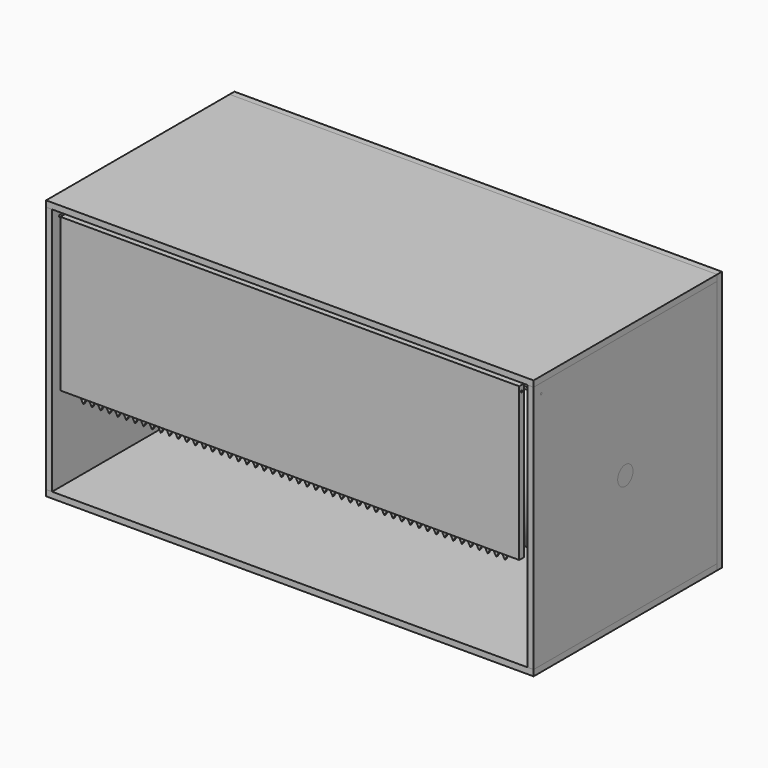
from build123d import *

# Parameters (mm, degrees)
F1_W           = 255
F1_H           = 120
F2_DEPTH       = 3.15
F3_W           = 120
F3_H           = 130
F4_DEPTH       = 3.15
F7_W           = 255
F7_H           = 136.3
F8_DEPTH       = 3.15
F11_R          = 42.8170068392
F11_R_2        = 11.8370629582
F12_DEPTH      = 115
F12_DEPTH_BACK = 115
F13_W          = 240
F13_H          = 80
F14_DEPTH      = 3.15
F16_DEPTH      = 1
F17_R          = 5
F17_R_2        = 0.5
F18_DEPTH      = 255.001
F19_R          = 5
F20_DEPTH      = 255
F19_R_2        = 0.5
F21_R          = 0.5
F22_DEPTH      = 247.501


with BuildPart() as f2:
    # F1 (on Top) → F2 (new body)
    with BuildSketch(Plane.XY):
        with Locations((127.5, 60)):
            Rectangle(F1_W, F1_H)
    extrude(amount=F2_DEPTH)


with BuildPart() as f4:
    # F3 (on face) → F4 (new body)
    with BuildSketch(Plane(origin=(0, 0, 0), x_dir=(0, -1, 0), z_dir=(-1, 0, 0))):
        with Locations((-60, 68.15)):
            Rectangle(F3_W, F3_H)
    extrude(amount=-F4_DEPTH)


with BuildPart() as f5_1:
    # F5: copy of F2
    add(f2.part.moved(Location((0, 0, 133.15))))


with BuildPart() as f6_1:
    # F6: copy of F4
    add(f4.part.moved(Location((251.85, 0, 0))))


with BuildPart() as f8:
    # F7 (on face) → F8 (new body)
    with BuildSketch(Plane(origin=(0, 120, 0), x_dir=(-1, 0, 0), z_dir=(0, 1, 0))):
        with Locations((-127.5, 68.15)):
            Rectangle(F7_W, F7_H)
    extrude(amount=F8_DEPTH)


with BuildPart() as f12:
    # F11 (on plane+point) → F12 (new body, two sides)
    with BuildSketch(Plane.YZ.offset(127.5)) as f12_sk:
        with Locations((62.5, 68.15)):
            Circle(F11_R)
        with Locations((62.5, 68.15)):
            Circle(F11_R_2, mode=Mode.SUBTRACT)
    extrude(amount=F12_DEPTH)
    extrude(f12_sk.sketch, amount=-F12_DEPTH_BACK)


with BuildPart() as f14:
    # F13 (on face) → F14 (new body)
    with BuildSketch(Plane.XZ):
        with Locations((127.5, 91.15)):
            Rectangle(F13_W, F13_H)
    extrude(amount=-F14_DEPTH)

    # F21 (on face) → F22 (cut, through all)
    with BuildSketch(Plane.YZ.offset(247.5)):
        with Locations((1.575, 128.15)):
            Circle(F21_R)
    extrude(amount=-F22_DEPTH, mode=Mode.SUBTRACT)


with BuildPart() as f16:
    # F15 (on face) → F16 (new body)
    with BuildSketch(Plane(origin=(0, 3.15, 0), x_dir=(-1, 0, 0), z_dir=(0, 1, 0))):
        Polygon((-231.0417766441, 51.15), (-234.8456242214, 51.15), (-235.1937004328, 50.547114317), (-232.9437004328, 46.65), (-230.6937004328, 50.547114317), align=None)
        Polygon((-235.1937004328, 50.547114317), (-234.8456242214, 51.15), (-235.5417766441, 51.15), align=None)
        Polygon((-235.5417766441, 51.15), (-234.8456242214, 51.15), (-231.0417766441, 51.15), (-230.3456242214, 51.15), (-226.5417766441, 51.15), (-225.8456242214, 51.15), (-222.0417766441, 51.15), (-221.3456242214, 51.15), (-217.5417766441, 51.15), (-216.8456242214, 51.15), (-213.0417766441, 51.15), (-212.3456242214, 51.15), (-208.5417766441, 51.15), (-207.8456242214, 51.15), (-204.0417766441, 51.15), (-203.3456242214, 51.15), (-199.5417766441, 51.15), (-198.8456242214, 51.15), (-195.0417766441, 51.15), (-194.3456242214, 51.15), (-190.5417766441, 51.15), (-189.8456242214, 51.15), (-186.0417766441, 51.15), (-185.3456242214, 51.15), (-181.5417766441, 51.15), (-180.8456242214, 51.15), (-177.0417766441, 51.15), (-176.3456242214, 51.15), (-172.5417766441, 51.15), (-171.8456242214, 51.15), (-168.0417766441, 51.15), (-167.3456242214, 51.15), (-163.5417766441, 51.15), (-162.8456242214, 51.15), (-159.0417766441, 51.15), (-158.3456242214, 51.15), (-154.5417766441, 51.15), (-153.8456242214, 51.15), (-150.0417766441, 51.15), (-149.3456242214, 51.15), (-145.5417766441, 51.15), (-144.8456242214, 51.15), (-141.0417766441, 51.15), (-140.3456242214, 51.15), (-136.5417766441, 51.15), (-135.8456242214, 51.15), (-132.0417766441, 51.15), (-131.3456242214, 51.15), (-127.5417766441, 51.15), (-126.8456242214, 51.15), (-123.0417766441, 51.15), (-122.3456242214, 51.15), (-118.5417766441, 51.15), (-117.8456242214, 51.15), (-114.0417766441, 51.15), (-113.3456242214, 51.15), (-109.5417766441, 51.15), (-108.8456242214, 51.15), (-105.0417766441, 51.15), (-104.3456242214, 51.15), (-100.5417766441, 51.15), (-99.8456242214, 51.15), (-96.0417766441, 51.15), (-95.3456242214, 51.15), (-91.5417766441, 51.15), (-90.8456242214, 51.15), (-87.0417766441, 51.15), (-86.3456242214, 51.15), (-82.5417766441, 51.15), (-81.8456242214, 51.15), (-78.0417766441, 51.15), (-77.3456242214, 51.15), (-73.5417766441, 51.15), (-72.8456242214, 51.15), (-69.0417766441, 51.15), (-68.3456242214, 51.15), (-64.5417766441, 51.15), (-63.8456242214, 51.15), (-60.0417766441, 51.15), (-59.3456242214, 51.15), (-55.5417766441, 51.15), (-54.8456242214, 51.15), (-51.0417766441, 51.15), (-50.3456242214, 51.15), (-46.5417766441, 51.15), (-45.8456242214, 51.15), (-42.0417766441, 51.15), (-41.3456242214, 51.15), (-37.5417766441, 51.15), (-36.8456242214, 51.15), (-33.0417766441, 51.15), (-32.3456242214, 51.15), (-28.5417766441, 51.15), (-27.8456242214, 51.15), (-24.0417766441, 51.15), (-23.3456242214, 51.15), (-19.5417766441, 51.15), (-18.8456242214, 51.15), (-14.3456242214, 51.15), (-14.3456242214, 56.283839047), (-240.0417766441, 56.283839047), (-240.0417766441, 51.15), align=None)
        Polygon((-237.4437004328, 46.65), (-235.1937004328, 50.547114317), (-235.5417766441, 51.15), (-240.0417766441, 51.15), align=None)
        Polygon((-230.3456242214, 51.15), (-231.0417766441, 51.15), (-230.6937004328, 50.547114317), align=None)
        Polygon((-226.5417766441, 51.15), (-230.3456242214, 51.15), (-230.6937004328, 50.547114317), (-228.4437004328, 46.65), (-226.1937004328, 50.547114317), align=None)
        Polygon((-225.8456242214, 51.15), (-226.5417766441, 51.15), (-226.1937004328, 50.547114317), align=None)
        Polygon((-222.0417766441, 51.15), (-225.8456242214, 51.15), (-226.1937004328, 50.547114317), (-223.9437004328, 46.65), (-221.6937004328, 50.547114317), align=None)
        Polygon((-16.9437004328, 46.65), (-14.3456242214, 51.15), (-18.8456242214, 51.15), (-19.1937004328, 50.547114317), align=None)
        Polygon((-221.3456242214, 51.15), (-222.0417766441, 51.15), (-221.6937004328, 50.547114317), align=None)
        Polygon((-19.1937004328, 50.547114317), (-18.8456242214, 51.15), (-19.5417766441, 51.15), align=None)
        Polygon((-217.5417766441, 51.15), (-221.3456242214, 51.15), (-221.6937004328, 50.547114317), (-219.4437004328, 46.65), (-217.1937004328, 50.547114317), align=None)
        Polygon((-21.4437004328, 46.65), (-19.1937004328, 50.547114317), (-19.5417766441, 51.15), (-23.3456242214, 51.15), (-23.6937004328, 50.547114317), align=None)
        Polygon((-216.8456242214, 51.15), (-217.5417766441, 51.15), (-217.1937004328, 50.547114317), align=None)
        Polygon((-23.6937004328, 50.547114317), (-23.3456242214, 51.15), (-24.0417766441, 51.15), align=None)
        Polygon((-213.0417766441, 51.15), (-216.8456242214, 51.15), (-217.1937004328, 50.547114317), (-214.9437004328, 46.65), (-212.6937004328, 50.547114317), align=None)
        Polygon((-25.9437004328, 46.65), (-23.6937004328, 50.547114317), (-24.0417766441, 51.15), (-27.8456242214, 51.15), (-28.1937004328, 50.547114317), align=None)
        Polygon((-212.3456242214, 51.15), (-213.0417766441, 51.15), (-212.6937004328, 50.547114317), align=None)
        Polygon((-28.1937004328, 50.547114317), (-27.8456242214, 51.15), (-28.5417766441, 51.15), align=None)
        Polygon((-208.5417766441, 51.15), (-212.3456242214, 51.15), (-212.6937004328, 50.547114317), (-210.4437004328, 46.65), (-208.1937004328, 50.547114317), align=None)
        Polygon((-30.4437004328, 46.65), (-28.1937004328, 50.547114317), (-28.5417766441, 51.15), (-32.3456242214, 51.15), (-32.6937004328, 50.547114317), align=None)
        Polygon((-207.8456242214, 51.15), (-208.5417766441, 51.15), (-208.1937004328, 50.547114317), align=None)
        Polygon((-32.6937004328, 50.547114317), (-32.3456242214, 51.15), (-33.0417766441, 51.15), align=None)
        Polygon((-204.0417766441, 51.15), (-207.8456242214, 51.15), (-208.1937004328, 50.547114317), (-205.9437004328, 46.65), (-203.6937004328, 50.547114317), align=None)
        Polygon((-34.9437004328, 46.65), (-32.6937004328, 50.547114317), (-33.0417766441, 51.15), (-36.8456242214, 51.15), (-37.1937004328, 50.547114317), align=None)
        Polygon((-203.3456242214, 51.15), (-204.0417766441, 51.15), (-203.6937004328, 50.547114317), align=None)
        Polygon((-37.1937004328, 50.547114317), (-36.8456242214, 51.15), (-37.5417766441, 51.15), align=None)
        Polygon((-199.5417766441, 51.15), (-203.3456242214, 51.15), (-203.6937004328, 50.547114317), (-201.4437004328, 46.65), (-199.1937004328, 50.547114317), align=None)
        Polygon((-39.4437004328, 46.65), (-37.1937004328, 50.547114317), (-37.5417766441, 51.15), (-41.3456242214, 51.15), (-41.6937004328, 50.547114317), align=None)
        Polygon((-198.8456242214, 51.15), (-199.5417766441, 51.15), (-199.1937004328, 50.547114317), align=None)
        Polygon((-41.6937004328, 50.547114317), (-41.3456242214, 51.15), (-42.0417766441, 51.15), align=None)
        Polygon((-195.0417766441, 51.15), (-198.8456242214, 51.15), (-199.1937004328, 50.547114317), (-196.9437004328, 46.65), (-194.6937004328, 50.547114317), align=None)
        Polygon((-43.9437004328, 46.65), (-41.6937004328, 50.547114317), (-42.0417766441, 51.15), (-45.8456242214, 51.15), (-46.1937004328, 50.547114317), align=None)
        Polygon((-194.3456242214, 51.15), (-195.0417766441, 51.15), (-194.6937004328, 50.547114317), align=None)
        Polygon((-46.1937004328, 50.547114317), (-45.8456242214, 51.15), (-46.5417766441, 51.15), align=None)
        Polygon((-190.5417766441, 51.15), (-194.3456242214, 51.15), (-194.6937004328, 50.547114317), (-192.4437004328, 46.65), (-190.1937004328, 50.547114317), align=None)
        Polygon((-48.4437004328, 46.65), (-46.1937004328, 50.547114317), (-46.5417766441, 51.15), (-50.3456242214, 51.15), (-50.6937004328, 50.547114317), align=None)
        Polygon((-189.8456242214, 51.15), (-190.5417766441, 51.15), (-190.1937004328, 50.547114317), align=None)
        Polygon((-50.6937004328, 50.547114317), (-50.3456242214, 51.15), (-51.0417766441, 51.15), align=None)
        Polygon((-186.0417766441, 51.15), (-189.8456242214, 51.15), (-190.1937004328, 50.547114317), (-187.9437004328, 46.65), (-185.6937004328, 50.547114317), align=None)
        Polygon((-52.9437004328, 46.65), (-50.6937004328, 50.547114317), (-51.0417766441, 51.15), (-54.8456242214, 51.15), (-55.1937004328, 50.547114317), align=None)
        Polygon((-185.3456242214, 51.15), (-186.0417766441, 51.15), (-185.6937004328, 50.547114317), align=None)
        Polygon((-55.1937004328, 50.547114317), (-54.8456242214, 51.15), (-55.5417766441, 51.15), align=None)
        Polygon((-181.5417766441, 51.15), (-185.3456242214, 51.15), (-185.6937004328, 50.547114317), (-183.4437004328, 46.65), (-181.1937004328, 50.547114317), align=None)
        Polygon((-57.4437004328, 46.65), (-55.1937004328, 50.547114317), (-55.5417766441, 51.15), (-59.3456242214, 51.15), (-59.6937004328, 50.547114317), align=None)
        Polygon((-180.8456242214, 51.15), (-181.5417766441, 51.15), (-181.1937004328, 50.547114317), align=None)
        Polygon((-59.6937004328, 50.547114317), (-59.3456242214, 51.15), (-60.0417766441, 51.15), align=None)
        Polygon((-177.0417766441, 51.15), (-180.8456242214, 51.15), (-181.1937004328, 50.547114317), (-178.9437004328, 46.65), (-176.6937004328, 50.547114317), align=None)
        Polygon((-61.9437004328, 46.65), (-59.6937004328, 50.547114317), (-60.0417766441, 51.15), (-63.8456242214, 51.15), (-64.1937004328, 50.547114317), align=None)
        Polygon((-176.3456242214, 51.15), (-177.0417766441, 51.15), (-176.6937004328, 50.547114317), align=None)
        Polygon((-64.1937004328, 50.547114317), (-63.8456242214, 51.15), (-64.5417766441, 51.15), align=None)
        Polygon((-172.5417766441, 51.15), (-176.3456242214, 51.15), (-176.6937004328, 50.547114317), (-174.4437004328, 46.65), (-172.1937004328, 50.547114317), align=None)
        Polygon((-66.4437004328, 46.65), (-64.1937004328, 50.547114317), (-64.5417766441, 51.15), (-68.3456242214, 51.15), (-68.6937004328, 50.547114317), align=None)
        Polygon((-171.8456242214, 51.15), (-172.5417766441, 51.15), (-172.1937004328, 50.547114317), align=None)
        Polygon((-68.6937004328, 50.547114317), (-68.3456242214, 51.15), (-69.0417766441, 51.15), align=None)
        Polygon((-168.0417766441, 51.15), (-171.8456242214, 51.15), (-172.1937004328, 50.547114317), (-169.9437004328, 46.65), (-167.6937004328, 50.547114317), align=None)
        Polygon((-70.9437004328, 46.65), (-68.6937004328, 50.547114317), (-69.0417766441, 51.15), (-72.8456242214, 51.15), (-73.1937004328, 50.547114317), align=None)
        Polygon((-167.3456242214, 51.15), (-168.0417766441, 51.15), (-167.6937004328, 50.547114317), align=None)
        Polygon((-73.1937004328, 50.547114317), (-72.8456242214, 51.15), (-73.5417766441, 51.15), align=None)
        Polygon((-163.5417766441, 51.15), (-167.3456242214, 51.15), (-167.6937004328, 50.547114317), (-165.4437004328, 46.65), (-163.1937004328, 50.547114317), align=None)
        Polygon((-75.4437004328, 46.65), (-73.1937004328, 50.547114317), (-73.5417766441, 51.15), (-77.3456242214, 51.15), (-77.6937004328, 50.547114317), align=None)
        Polygon((-162.8456242214, 51.15), (-163.5417766441, 51.15), (-163.1937004328, 50.547114317), align=None)
        Polygon((-77.6937004328, 50.547114317), (-77.3456242214, 51.15), (-78.0417766441, 51.15), align=None)
        Polygon((-159.0417766441, 51.15), (-162.8456242214, 51.15), (-163.1937004328, 50.547114317), (-160.9437004328, 46.65), (-158.6937004328, 50.547114317), align=None)
        Polygon((-79.9437004328, 46.65), (-77.6937004328, 50.547114317), (-78.0417766441, 51.15), (-81.8456242214, 51.15), (-82.1937004328, 50.547114317), align=None)
        Polygon((-158.3456242214, 51.15), (-159.0417766441, 51.15), (-158.6937004328, 50.547114317), align=None)
        Polygon((-82.1937004328, 50.547114317), (-81.8456242214, 51.15), (-82.5417766441, 51.15), align=None)
        Polygon((-154.5417766441, 51.15), (-158.3456242214, 51.15), (-158.6937004328, 50.547114317), (-156.4437004328, 46.65), (-154.1937004328, 50.547114317), align=None)
        Polygon((-84.4437004328, 46.65), (-82.1937004328, 50.547114317), (-82.5417766441, 51.15), (-86.3456242214, 51.15), (-86.6937004328, 50.547114317), align=None)
        Polygon((-153.8456242214, 51.15), (-154.5417766441, 51.15), (-154.1937004328, 50.547114317), align=None)
        Polygon((-86.6937004328, 50.547114317), (-86.3456242214, 51.15), (-87.0417766441, 51.15), align=None)
        Polygon((-150.0417766441, 51.15), (-153.8456242214, 51.15), (-154.1937004328, 50.547114317), (-151.9437004328, 46.65), (-149.6937004328, 50.547114317), align=None)
        Polygon((-88.9437004328, 46.65), (-86.6937004328, 50.547114317), (-87.0417766441, 51.15), (-90.8456242214, 51.15), (-91.1937004328, 50.547114317), align=None)
        Polygon((-149.3456242214, 51.15), (-150.0417766441, 51.15), (-149.6937004328, 50.547114317), align=None)
        Polygon((-91.1937004328, 50.547114317), (-90.8456242214, 51.15), (-91.5417766441, 51.15), align=None)
        Polygon((-145.5417766441, 51.15), (-149.3456242214, 51.15), (-149.6937004328, 50.547114317), (-147.4437004328, 46.65), (-145.1937004328, 50.547114317), align=None)
        Polygon((-93.4437004328, 46.65), (-91.1937004328, 50.547114317), (-91.5417766441, 51.15), (-95.3456242214, 51.15), (-95.6937004328, 50.547114317), align=None)
        Polygon((-144.8456242214, 51.15), (-145.5417766441, 51.15), (-145.1937004328, 50.547114317), align=None)
        Polygon((-95.6937004328, 50.547114317), (-95.3456242214, 51.15), (-96.0417766441, 51.15), align=None)
        Polygon((-141.0417766441, 51.15), (-144.8456242214, 51.15), (-145.1937004328, 50.547114317), (-142.9437004328, 46.65), (-140.6937004328, 50.547114317), align=None)
        Polygon((-97.9437004328, 46.65), (-95.6937004328, 50.547114317), (-96.0417766441, 51.15), (-99.8456242214, 51.15), (-100.1937004328, 50.547114317), align=None)
        Polygon((-140.3456242214, 51.15), (-141.0417766441, 51.15), (-140.6937004328, 50.547114317), align=None)
        Polygon((-100.1937004328, 50.547114317), (-99.8456242214, 51.15), (-100.5417766441, 51.15), align=None)
        Polygon((-136.5417766441, 51.15), (-140.3456242214, 51.15), (-140.6937004328, 50.547114317), (-138.4437004328, 46.65), (-136.1937004328, 50.547114317), align=None)
        Polygon((-102.4437004328, 46.65), (-100.1937004328, 50.547114317), (-100.5417766441, 51.15), (-104.3456242214, 51.15), (-104.6937004328, 50.547114317), align=None)
        Polygon((-135.8456242214, 51.15), (-136.5417766441, 51.15), (-136.1937004328, 50.547114317), align=None)
        Polygon((-104.6937004328, 50.547114317), (-104.3456242214, 51.15), (-105.0417766441, 51.15), align=None)
        Polygon((-132.0417766441, 51.15), (-135.8456242214, 51.15), (-136.1937004328, 50.547114317), (-133.9437004328, 46.65), (-131.6937004328, 50.547114317), align=None)
        Polygon((-106.9437004328, 46.65), (-104.6937004328, 50.547114317), (-105.0417766441, 51.15), (-108.8456242214, 51.15), (-109.1937004328, 50.547114317), align=None)
        Polygon((-131.3456242214, 51.15), (-132.0417766441, 51.15), (-131.6937004328, 50.547114317), align=None)
        Polygon((-109.1937004328, 50.547114317), (-108.8456242214, 51.15), (-109.5417766441, 51.15), align=None)
        Polygon((-127.5417766441, 51.15), (-131.3456242214, 51.15), (-131.6937004328, 50.547114317), (-129.4437004328, 46.65), (-127.1937004328, 50.547114317), align=None)
        Polygon((-111.4437004328, 46.65), (-109.1937004328, 50.547114317), (-109.5417766441, 51.15), (-113.3456242214, 51.15), (-113.6937004328, 50.547114317), align=None)
        Polygon((-126.8456242214, 51.15), (-127.5417766441, 51.15), (-127.1937004328, 50.547114317), align=None)
        Polygon((-113.6937004328, 50.547114317), (-113.3456242214, 51.15), (-114.0417766441, 51.15), align=None)
        Polygon((-123.0417766441, 51.15), (-126.8456242214, 51.15), (-127.1937004328, 50.547114317), (-124.9437004328, 46.65), (-122.6937004328, 50.547114317), align=None)
        Polygon((-115.9437004328, 46.65), (-113.6937004328, 50.547114317), (-114.0417766441, 51.15), (-117.8456242214, 51.15), (-118.1937004328, 50.547114317), align=None)
        Polygon((-122.3456242214, 51.15), (-123.0417766441, 51.15), (-122.6937004328, 50.547114317), align=None)
        Polygon((-118.1937004328, 50.547114317), (-117.8456242214, 51.15), (-118.5417766441, 51.15), align=None)
        Polygon((-118.5417766441, 51.15), (-122.3456242214, 51.15), (-122.6937004328, 50.547114317), (-120.4437004328, 46.65), (-118.1937004328, 50.547114317), align=None)
    extrude(amount=F16_DEPTH)


with BuildPart() as f18_tool:
    # F17 (on face) → F18 (new body, through all)
    with BuildSketch(Plane.YZ.offset(255)):
        with Locations((60, 68.15)):
            Circle(F17_R)
        with Locations((5, 128.15)):
            Circle(F17_R_2)
    extrude(amount=-F18_DEPTH)


with BuildPart() as f4_1:
    add(f4.part)

    # F18: cut by f18_tool
    add(f18_tool.part, mode=Mode.SUBTRACT)


with BuildPart() as f6_1_1:
    add(f6_1.part)

    # F18: cut by f18_tool
    add(f18_tool.part, mode=Mode.SUBTRACT)


with BuildPart() as f20:
    # F19 (on face) → F20 (new body, through all)
    with BuildSketch(Plane.YZ.offset(255)):
        with Locations((60, 68.15)):
            Circle(F19_R)
    extrude(amount=-F20_DEPTH)


with BuildPart() as f20b:
    # F19 (on face) → F20, piece 2 (new body, through all)
    with BuildSketch(Plane.YZ.offset(255)):
        with Locations((5, 128.15)):
            Circle(F19_R_2)
    extrude(amount=-F20_DEPTH)


solid = Compound([f2.part, f5_1.part, f8.part, f12.part, f14.part, f16.part, f4_1.part, f6_1_1.part, f20.part, f20b.part])
